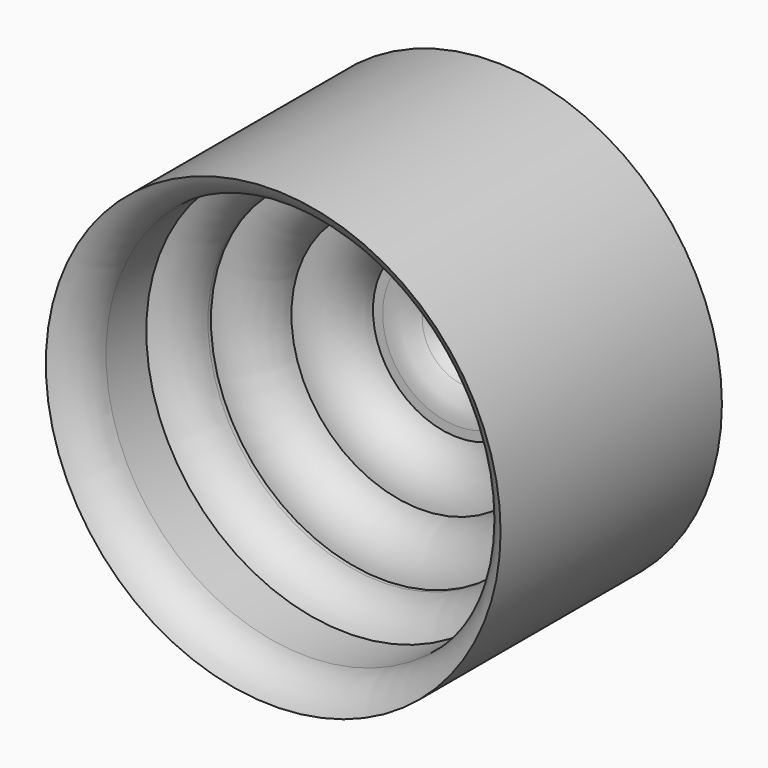
from build123d import *

# Parameters (mm, degrees)
F0_R     = 25.0538592269
F0_R_2   = 22.1151021615
F1_DEPTH = 30.48
F0_R_3   = 19.05
F2_DEPTH = 20.32
F0_R_4   = 14.2519488642
F3_DEPTH = 15.24
F0_R_5   = 9.329458502
F4_DEPTH = 10.16
F0_R_6   = 4.9036289707
F5_DEPTH = 5.08
F0_R_7   = 2.6620736833
F6_DEPTH = 3.81
F7_DEPTH = 15.24


# Not quite as in the source:
# - a fillet or chamfer that OpenCascade refuses, or shapes differently, is made with other operations: its cross-section is extruded or revolved along the edge and cut away or added


with BuildPart() as f1:
    # F0 (on Front) → F1 (new body)
    with BuildSketch(Plane.XZ):
        Circle(F0_R)
        Circle(F0_R_2, mode=Mode.SUBTRACT)
    extrude(amount=F1_DEPTH)

    # F0 (on Front) → F2 (join)
    with BuildSketch(Plane.XZ):
        Circle(F0_R_2)
        Circle(F0_R_3, mode=Mode.SUBTRACT)
    extrude(amount=F2_DEPTH)

    # F0 (on Front) → F3 (join)
    with BuildSketch(Plane.XZ):
        Circle(F0_R_3)
        Circle(F0_R_4, mode=Mode.SUBTRACT)
    extrude(amount=F3_DEPTH)

    # F0 (on Front) → F4 (join)
    with BuildSketch(Plane.XZ):
        Circle(F0_R_4)
        Circle(F0_R_5, mode=Mode.SUBTRACT)
    extrude(amount=F4_DEPTH)

    # F0 (on Front) → F5 (join)
    with BuildSketch(Plane.XZ):
        Circle(F0_R_5)
        Circle(F0_R_6, mode=Mode.SUBTRACT)
    extrude(amount=F5_DEPTH)

    # F0 (on Front) → F6 (join)
    with BuildSketch(Plane.XZ):
        Circle(F0_R_6)
        Circle(F0_R_7, mode=Mode.SUBTRACT)
    extrude(amount=F6_DEPTH)

    # F0 (on Front) → F7 (join)
    with BuildSketch(Plane.XZ):
        Circle(F0_R_6)
        Circle(F0_R_7, mode=Mode.SUBTRACT)
    extrude(amount=-F7_DEPTH)

    # F8: fillet of radius 5.08 on 6 edges, made by hand

    # F8_s1 → F8_t2 (revolve, cut)
    with BuildSketch(Plane.XY):
        with BuildLine():
            ThreePointArc((25.0538592269, -30.48), (22.9123510534, -28.6054356547), (22.1151021615, -25.87332238))
            Line((22.1151021615, -25.87332238), (22.1151021615, -30.48))
            Line((22.1151021615, -30.48), (25.0538592269, -30.48))
        make_face()
    revolve(axis=Axis((0, -30.48, 0), (0, -1, 0)), mode=Mode.SUBTRACT)

    # F8_s3 → F8_t4 (revolve, cut)
    with BuildSketch(Plane.XY):
        with BuildLine():
            ThreePointArc((22.1151021615, -20.32), (19.8848803892, -18.4469021379), (19.05, -15.6566764319))
            Line((19.05, -15.6566764319), (19.05, -20.32))
            Line((19.05, -20.32), (22.1151021615, -20.32))
        make_face()
    revolve(axis=Axis((0, -20.32, 0), (0, -1, 0)), mode=Mode.SUBTRACT)

    # F8_s5 → F8_t6 (revolve, cut)
    with BuildSketch(Plane.XY):
        with BuildLine():
            ThreePointArc((19.05, -15.24), (15.6415084955, -13.6588259054), (14.2519488642, -10.1678303619))
            Line((14.2519488642, -10.1678303619), (14.2519488642, -15.24))
            Line((14.2519488642, -15.24), (19.05, -15.24))
        make_face()
    revolve(axis=Axis((0, -15.24, 0), (0, -1, 0)), mode=Mode.SUBTRACT)

    # F8_s7 → F8_t8 (revolve, cut)
    with BuildSketch(Plane.XY):
        with BuildLine():
            ThreePointArc((14.2519488642, -10.16), (10.7620930857, -8.6184183396), (9.329458502, -5.082442446))
            Line((9.329458502, -5.082442446), (9.329458502, -10.16))
            Line((9.329458502, -10.16), (14.2519488642, -10.16))
        make_face()
    revolve(axis=Axis((0, -10.16, 0), (0, -1, 0)), mode=Mode.SUBTRACT)

    # F8_s9 → F8_t10 (revolve, cut)
    with BuildSketch(Plane.XY):
        with BuildLine():
            ThreePointArc((4.9036289707, -3.81), (6.4676819116, -4.7519048812), (8.2637331358, -5.08))
            Line((8.2637331358, -5.08), (4.9036289707, -5.08))
            Line((4.9036289707, -5.08), (4.9036289707, -3.81))
        make_face()
    revolve(axis=Axis((0, -5.08, 0), (0, -1, 0)), mode=Mode.SUBTRACT)

    # F8_s11 → F8_t12 (revolve, cut)
    with BuildSketch(Plane.XY):
        with BuildLine():
            ThreePointArc((2.6620736833, 0.4030311669), (3.2573385105, -1.9830850142), (4.9036289707, -3.81))
            Line((4.9036289707, -3.81), (2.6620736833, -3.81))
            Line((2.6620736833, -3.81), (2.6620736833, 0.4030311669))
        make_face()
    revolve(axis=Axis((0, -3.81, 0), (0, -1, 0)), mode=Mode.SUBTRACT)


solid = f1.part
